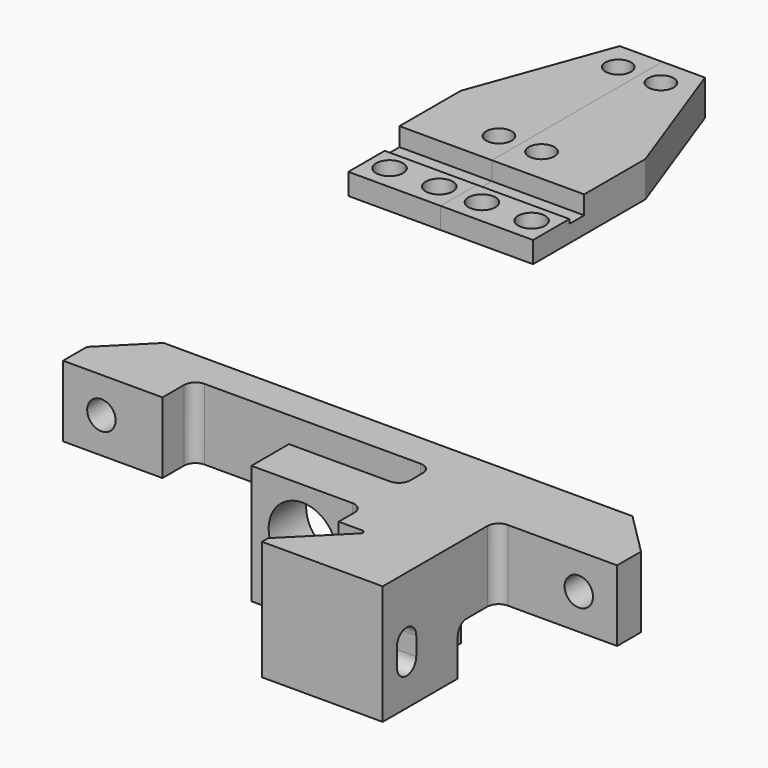
from build123d import *

# Parameters (mm, degrees)
F0_R         = 0.9
F1_DEPTH     = 2.5
F0_W         = 6.5
F0_H         = 1.3
F2_DEPTH     = 1.2
F0_H_2       = 3.2
F0_R_2       = 0.95
F3_DEPTH     = 1.5
F5_DEPTH     = 5
F6_DEPTH     = 8.4
F8_D         = 2
F8_DEPTH     = 14.4
F8_TIP       = 0.600860619
F10_DEPTH    = 3.8
F11_R        = 0.85
F12_DEPTH    = 30.501
F13_R        = 0.8
F14_T1_DEPTH = 20.4300979278
F15_R        = 0.2


# Not quite as in the source:
# - a fillet or chamfer that OpenCascade refuses, or shapes differently, is made with other operations: its cross-section is extruded or revolved along the edge and cut away or added


with BuildPart() as f1:
    # F0 (on Top) → F1 (new body)
    with BuildSketch(Plane.XY):
        Polygon((0, 9.8838290319), (0, 4.5), (6.5, 4.5), (6.5, 19.5), (3.5, 19.5), align=None)
        with Locations((5, 7)):
            Circle(F0_R, mode=Mode.SUBTRACT)
        with Locations((5, 17.5)):
            Circle(F0_R, mode=Mode.SUBTRACT)
    extrude(amount=F1_DEPTH)

    # F0 (on Top) → F2 (join)
    with BuildSketch(Plane.XY):
        with Locations((3.25, 3.85)):
            Rectangle(F0_W, F0_H)
    extrude(amount=F2_DEPTH)

    # F0 (on Top) → F3 (join)
    with BuildSketch(Plane.XY):
        with Locations((3.25, 1.6)):
            Rectangle(F0_W, F0_H_2)
        with Locations((1.5, 1.75)):
            Circle(F0_R_2, mode=Mode.SUBTRACT)
        with Locations((5, 1.75)):
            Circle(F0_R_2, mode=Mode.SUBTRACT)
    extrude(amount=F3_DEPTH)


with BuildPart() as f4_1:
    # F4: instance of F1
    add(f1.part.mirror(Plane(origin=(6.5, 10.5719562244, 1.1721614227), x_dir=(0, 1, 0), z_dir=(1, 0, 0))))


with BuildPart() as f5:
    # F0 (on Top) → F5 (new body)
    with BuildSketch(Plane.XY):
        Polygon((0, -20), (0, -25.1), (7, -25.1), (7, -22.4), (23.8, -22.4), (23.8, -25.1), (28, -25.1), (28, -28.5), (30.5, -28.5), (30.5, -25.1), (39, -25.1), (39, -20), align=None)
    extrude(amount=-F5_DEPTH)

    # F0 (on Top) → F6 (join)
    with BuildSketch(Plane.XY):
        Polygon((28, -25.1), (23.8, -25.1), (15.9, -25.1), (15.9, -28.4), (23.8, -28.4), (23.8, -30.6), (25.9500320151, -30.6), (22, -34.5500320151), (22, -35.1), (30.5, -35.1), (30.5, -28.5), (28, -28.5), align=None)
    extrude(amount=-F6_DEPTH)

    # F8
    with Locations(Plane(origin=(0, -20, 0), x_dir=(-1, 0, 0), z_dir=(0, 1, 0))):
        with Locations((-2.7, -2.5), (-36.3, -2.5)):
            Hole(F8_D / 2, depth=F8_DEPTH)
            with Locations((0, 0, -(F8_DEPTH + F8_TIP / 2))):  # 118° drill point
                Cone(0, F8_D / 2, F8_TIP, mode=Mode.SUBTRACT)

    # F9 (on face) → F10 (cut)
    with BuildSketch(Plane.XZ.offset(28.4)):
        with BuildLine():
            ThreePointArc((19.75, -5.8768887227), (21.276175667, -5.0991560274), (21.89, -3.5))
            ThreePointArc((21.89, -3.5), (17.9008439726, -1.723824333), (19.25, -5.8768887227))
            Line((19.25, -5.8768887227), (19.75, -5.8768887227))
        make_face()
        with BuildLine():
            ThreePointArc((19.75, -5.8768887227), (19.5, -5.89), (19.25, -5.8768887227))
            Line((19.25, -5.8768887227), (19.25, -8.4))
            Line((19.25, -8.4), (19.75, -8.4))
            Line((19.75, -8.4), (19.75, -5.8768887227))
        make_face()
        with BuildLine():
            Line((19.75, -5.8768887227), (19.25, -5.8768887227))
            ThreePointArc((19.25, -5.8768887227), (19.5, -5.89), (19.75, -5.8768887227))
        make_face()
    extrude(amount=-F10_DEPTH, mode=Mode.SUBTRACT)

    # F11 (on face) → F12 (cut, through all)
    with BuildSketch(Plane.YZ.offset(30.5)):
        with Locations((-26.8, -6.7)):
            Circle(F11_R)
        with BuildLine():
            Line((-33.85, -4.25), (-32.15, -4.25))
            ThreePointArc((-32.15, -4.25), (-33, -3.4), (-33.85, -4.25))
        make_face()
        with BuildLine():
            ThreePointArc((-32.4522774425, -4.9), (-32.2292652292, -4.6084242083), (-32.15, -4.25))
            Line((-32.15, -4.25), (-33.85, -4.25))
            ThreePointArc((-33.85, -4.25), (-33.7707347708, -4.6084242083), (-33.5477225575, -4.9))
            ThreePointArc((-33.5477225575, -4.9), (-33, -4.7), (-32.4522774425, -4.9))
        make_face()
        with BuildLine():
            Line((-33.85, -4.25), (-33.85, -5.55))
            ThreePointArc((-33.85, -5.55), (-33.7707347708, -5.1915757917), (-33.5477225575, -4.9))
            ThreePointArc((-33.5477225575, -4.9), (-33.7707347708, -4.6084242083), (-33.85, -4.25))
        make_face()
        with BuildLine():
            Line((-33.85, -5.55), (-32.15, -5.55))
            ThreePointArc((-32.15, -5.55), (-32.2292652292, -5.1915757917), (-32.4522774425, -4.9))
            ThreePointArc((-32.4522774425, -4.9), (-33, -5.1), (-33.5477225575, -4.9))
            ThreePointArc((-33.5477225575, -4.9), (-33.7707347708, -5.1915757917), (-33.85, -5.55))
        make_face()
        with BuildLine():
            ThreePointArc((-33.5477225575, -4.9), (-33, -5.1), (-32.4522774425, -4.9))
            ThreePointArc((-32.4522774425, -4.9), (-33, -4.7), (-33.5477225575, -4.9))
        make_face()
        with BuildLine():
            ThreePointArc((-32.4522774425, -4.9), (-32.2292652292, -5.1915757917), (-32.15, -5.55))
            Line((-32.15, -5.55), (-32.15, -4.25))
            ThreePointArc((-32.15, -4.25), (-32.2292652292, -4.6084242083), (-32.4522774425, -4.9))
        make_face()
        with BuildLine():
            ThreePointArc((-33.85, -5.55), (-33, -6.4), (-32.15, -5.55))
            Line((-32.15, -5.55), (-33.85, -5.55))
        make_face()
    extrude(amount=-F12_DEPTH, mode=Mode.SUBTRACT)

    # F13
    f13_edges = [f5.edges().sort_by_distance(p)[0] for p in [
        (29.25, -28.5, -5),
        (7, -22.4, -2.5),
        (23.8, -22.4, -2.5),
        (23.8, -25.1, -2.5),
        (30.5, -25.1, -2.5),
        (23.8, -28.4, -4.2),
    ]]
    fillet(f13_edges, radius=F13_R)

    # F14: chamfer of 3 on 2 edges, made by hand

    # F14_s2 → F14_t1 (cut)
    with BuildSketch(Plane.XY.offset(-12.7150489639)):
        Polygon((0, -23), (3, -20), (0, -20), align=None)
        Polygon((36, -20), (39, -23), (39, -20), align=None)
    extrude(amount=F14_T1_DEPTH, mode=Mode.SUBTRACT)

    # F15
    f15_edges = [f5.edges().sort_by_distance(p)[0] for p in [
        (25.950032, -30.6, -4.2),
    ]]
    fillet(f15_edges, radius=F15_R)


solid = Compound([f1.part, f4_1.part, f5.part])
